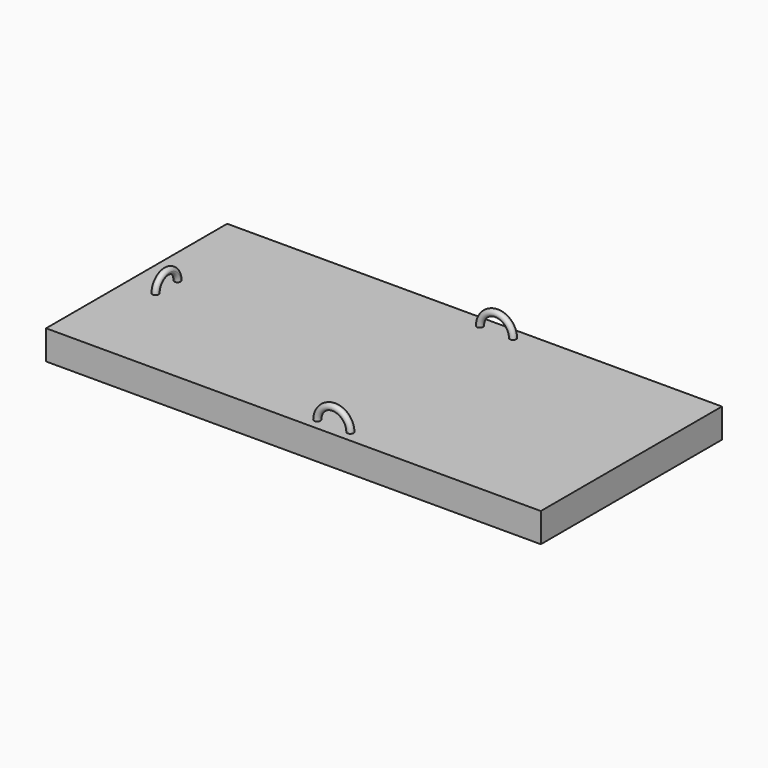
from build123d import *

# Parameters (mm, degrees)
F0_W     = 98.806
F0_H     = 45.212
F1_DEPTH = 2.921
F3_ANGLE = 180
F6_R     = 0.635


# Not quite as in the source:
# - the program builds the solid bodies; features that only make, move or delete a surface that nothing else refers to are left out


with BuildPart() as f1:
    # F0 (on Top) → F1 (new body, symmetric)
    with BuildSketch(Plane.XY):
        Rectangle(F0_W, F0_H)
    extrude(amount=F1_DEPTH, both=True)

    # F2 (on face) → F3 (revolve)
    with BuildSketch(Plane.XY.offset(2.921)):
        with BuildLine():
            ThreePointArc((-43.4750802815, 2.159), (-43.0260674754, 2.3449871939), (-42.8400802815, 2.794))
            ThreePointArc((-42.8400802815, 2.794), (-43.9240930875, 3.2430128061), (-43.4750802815, 2.159))
        make_face()
        with BuildLine():
            ThreePointArc((-42.8400802815, -2.6924), (-43.0260674754, -2.2433871939), (-43.4750802815, -2.0574))
            ThreePointArc((-43.4750802815, -2.0574), (-43.9240930875, -3.1414128061), (-42.8400802815, -2.6924))
        make_face()
    revolve(axis=Axis((-43.6497014016, 0.0508, 2.921), (-1, 0, 0)), revolution_arc=F3_ANGLE)

    # F6 (on face) → F7 (revolve)
    with BuildSketch(Plane.XY.offset(2.921)):
        with Locations((2.921, -20.3025657684)):
            Circle(F6_R)
        with BuildLine():
            ThreePointArc((10.16, -20.3025657684), (9.525, -19.6675657684), (8.89, -20.3025657684))
            ThreePointArc((8.89, -20.3025657684), (9.525, -20.9375657684), (10.16, -20.3025657684))
        make_face()
        with Locations((2.921, 20.3025657684)):
            Circle(F6_R)
        with BuildLine():
            ThreePointArc((10.16, 20.3025657684), (9.525, 20.9375657684), (8.89, 20.3025657684))
            ThreePointArc((8.89, 20.3025657684), (9.525, 19.6675657684), (10.16, 20.3025657684))
        make_face()
    revolve(axis=Axis((6.223, -20.2974760905, 2.921), (0, 1, 0)))


solid = f1.part
